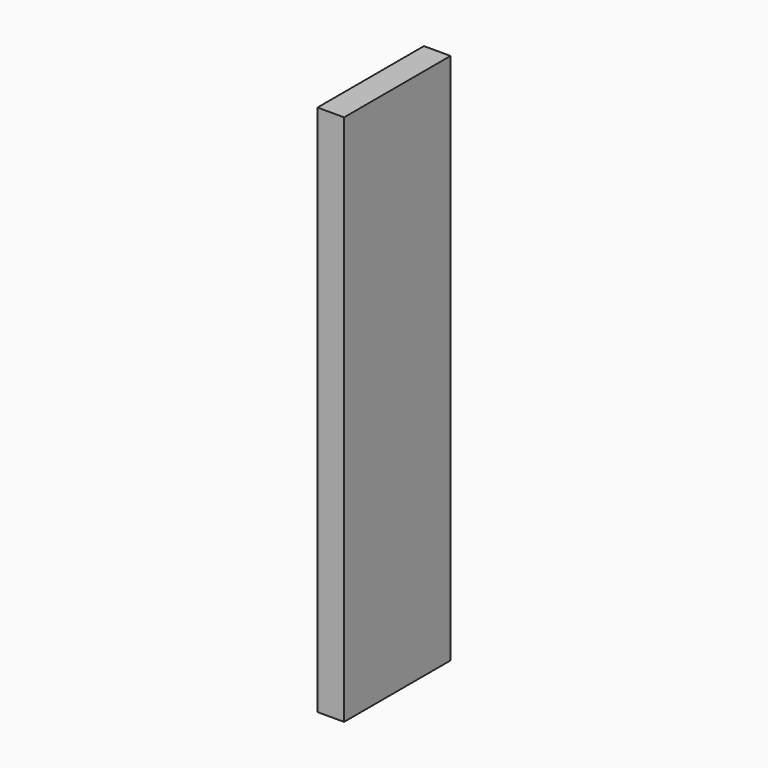
from build123d import *

# Parameters (mm, degrees)
F1_DEPTH = 1


# Not quite as in the source:
# - a feature of the source that left no trace in its solid (it failed there, or was rolled back) is left out


with BuildPart() as f1:
    # F0 (on Right) → F1 (new body, symmetric)
    with BuildSketch(Plane.YZ):
        Polygon((-35, -5), (-25, -5), (-25, 0), (-25, 35), (-35, 35), align=None)
    extrude(amount=F1_DEPTH, both=True)


solid = f1.part
